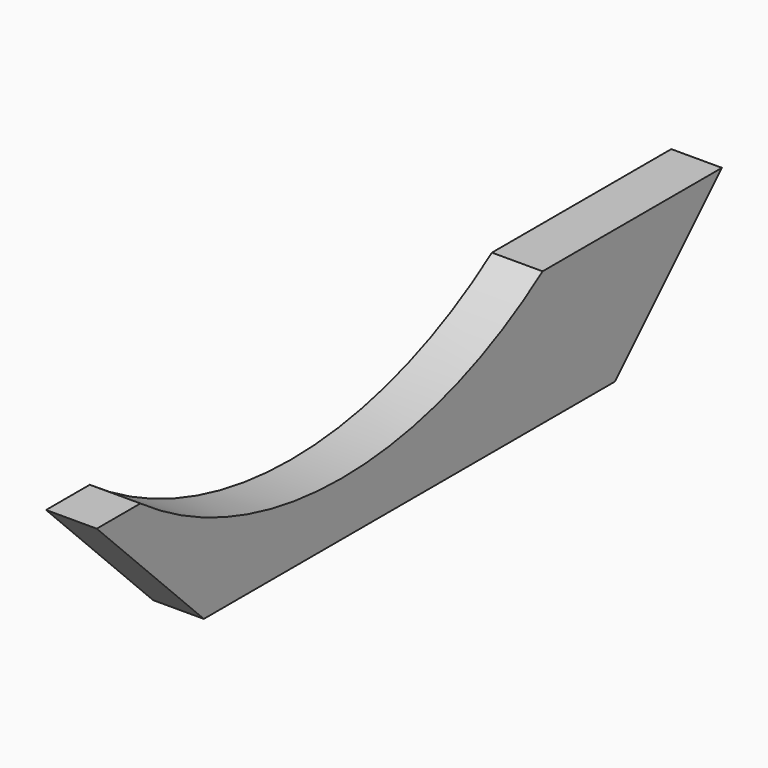
from build123d import *

# Parameters (mm, degrees)
F0_W     = 88.9
F0_H     = 234.95
F1_DEPTH = 685.8
F2_SIZE  = 234.94999
F3_SIZE  = 234.94999
F5_D     = 1524


# Not quite as in the source:
# - a fillet or chamfer is up to 0.001 mm smaller than in the source, because OpenCascade refuses the exact size


with BuildPart() as f1:
    # F0 (on Front) → F1 (new body, symmetric)
    with BuildSketch(Plane.XZ):
        Rectangle(F0_W, F0_H)
    extrude(amount=F1_DEPTH, both=True)

    # F2 (size 234.95 in the source; OpenCascade refuses exactly that, so slightly less here)
    f2_edges = [f1.edges().sort_by_distance(p)[0] for p in [
        (0, -685.8, -117.475),
    ]]
    chamfer(f2_edges, length=F2_SIZE)

    # F3 (size 234.95 in the source; OpenCascade refuses exactly that, so slightly less here)
    f3_edges = [f1.edges().sort_by_distance(p)[0] for p in [
        (0, 685.8, -117.475),
    ]]
    chamfer(f3_edges, length=F3_SIZE)

    # F5 (through all)
    with Locations(Plane(origin=(-44.45, 0, 0), x_dir=(0, -1, 0), z_dir=(-1, 0, 0))):
        with Locations((148.8177627325, 738.7712001801)):
            Hole(F5_D / 2)


solid = f1.part
